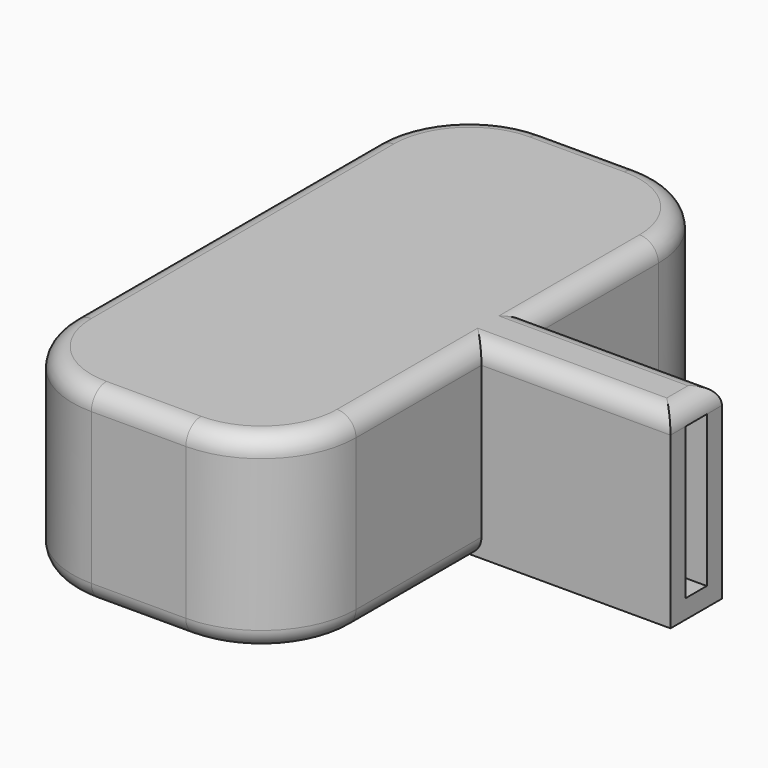
from build123d import *

# Parameters (mm, degrees)
F0_W     = 15
F0_H     = 30
F1_DEPTH = 10
F2_W     = 3.4
F2_H     = 10
F2_W_2   = 1.4
F2_H_2   = 8
F3_DEPTH = 10
F4_R     = 5
F5_R     = 1
F6_R     = 0.99999


# Not quite as in the source:
# - a fillet or chamfer is up to 0.001 mm smaller than in the source, because OpenCascade refuses the exact size


with BuildPart() as f1:
    # F0 (on Top) → F1 (new body)
    with BuildSketch(Plane.XY):
        with Locations((-25.6027433276, 15)):
            Rectangle(F0_W, F0_H)
    extrude(amount=F1_DEPTH)

    # F2 (on face) → F3 (join)
    with BuildSketch(Plane.YZ.offset(-18.1027433276)):
        with Locations((15, 5)):
            Rectangle(F2_W, F2_H)
        with Locations((15, 5)):
            Rectangle(F2_W_2, F2_H_2, mode=Mode.SUBTRACT)
    extrude(amount=F3_DEPTH)

    # F4
    f4_edges = [f1.edges().sort_by_distance(p)[0] for p in [
        (-18.102743, 30, 5),
        (-33.102743, 30, 5),
        (-33.102743, 0, 5),
        (-18.102743, 0, 5),
    ]]
    fillet(f4_edges, radius=F4_R)

    # F5
    f5_edges = [f1.edges().sort_by_distance(p)[0] for p in [
        (-33.102743, 15, 10),
        (-31.638277, 28.535534, 10),
        (-25.602743, 30, 10),
        (-19.567209, 28.535534, 10),
        (-18.102743, 20.85, 10),
        (-18.102743, 9.15, 10),
        (-19.567209, 1.464466, 10),
        (-25.602743, 0, 10),
        (-31.638277, 1.464466, 10),
    ]]
    fillet(f5_edges, radius=F5_R)

    # F6 (radius 1 in the source; OpenCascade refuses exactly that, so slightly less here)
    f6_edges = [f1.edges().sort_by_distance(p)[0] for p in [
        (-18.102743, 20.85, 0),
        (-18.102743, 9.15, 0),
        (-19.567209, 1.464466, 0),
        (-25.602743, 0, 0),
        (-31.638277, 1.464466, 0),
        (-33.102743, 15, 0),
        (-31.638277, 28.535534, 0),
        (-25.602743, 30, 0),
        (-19.567209, 28.535534, 0),
        (-18.602743, 16.7, 10),
        (-13.102743, 16.7, 10),
        (-19.102743, 20.85, 10),
        (-8.102743, 15, 10),
        (-20.274316, 27.828427, 10),
        (-13.102743, 13.3, 10),
        (-25.602743, 29, 10),
        (-18.602743, 13.3, 10),
        (-30.93117, 27.828427, 10),
        (-19.102743, 9.15, 10),
        (-32.102743, 15, 10),
        (-20.274316, 2.171573, 10),
        (-30.93117, 2.171573, 10),
        (-25.602743, 1, 10),
    ]]
    fillet(f6_edges, radius=F6_R)


solid = f1.part
